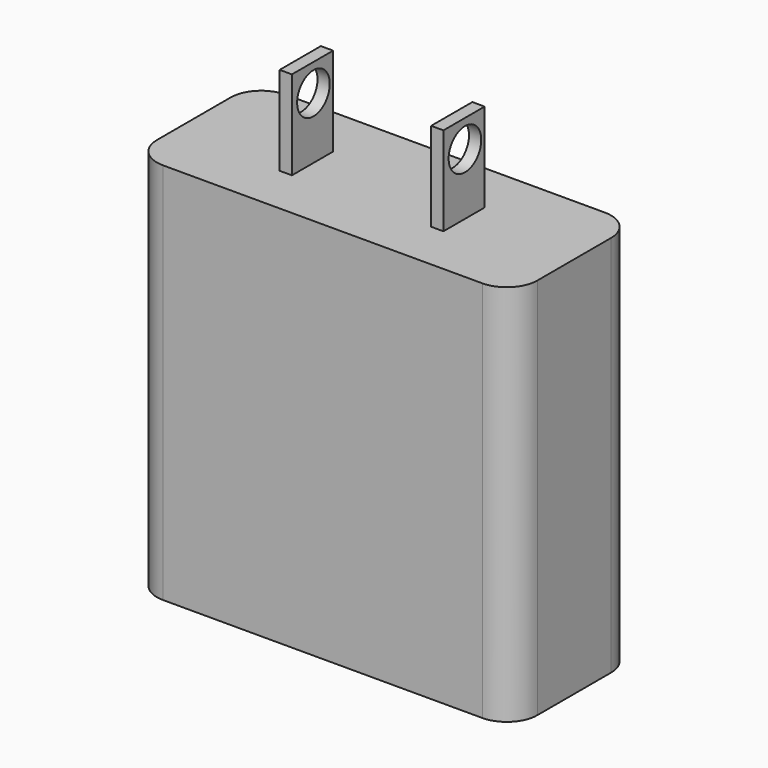
from build123d import *

# Parameters (mm, degrees)
F0_W      = 63.0582608283
F0_H      = 63.4325034916
F1_DEPTH  = 12.7
F2_R      = 5.08
F4_E1_W   = 8.5344002582
F4_E1_H   = 14.732
F5_DEPTH  = 2.032
F4_E2_W   = 8.5344002582
F4_E2_H   = 14.732
F6_DEPTH  = 2.032
F8_D      = 6.7564
F9_W      = 11.2923893612
F9_H      = 4.2961570434
F10_DEPTH = 7.112
F11_R     = 1.4717045876


with BuildPart() as f1:
    # F0 (on Front) → F1 (new body, symmetric)
    with BuildSketch(Plane.XZ):
        with Locations((-4.5010391623, -6.8866405636)):
            Rectangle(F0_W, F0_H)
    extrude(amount=F1_DEPTH, both=True)

    # F2
    f2_edges = [f1.edges().sort_by_distance(p)[0] for p in [
        (27.028091, -12.7, -6.886641),
        (27.028091, 12.7, -6.886641),
        (-36.03017, 12.7, -6.886641),
        (-36.03017, -12.7, -6.886641),
    ]]
    fillet(f2_edges, radius=F2_R)

    # F4_E1 (on explicit) → F5 (join)
    with BuildSketch(Plane(origin=(-16.1959640682, 4.0732366033, 24.8296111822), x_dir=(0, -1, 0), z_dir=(-1, 0, 0))):
        with Locations((4.2672001291, 7.366)):
            Rectangle(F4_E1_W, F4_E1_H)
    extrude(amount=F5_DEPTH)

    # F4_E2 (on explicit) → F6 (join)
    with BuildSketch(Plane(origin=(6.8857083097, 4.0732364287, 24.8296111822), x_dir=(0, -1, 0), z_dir=(-1, 0, 0))):
        with Locations((4.2672001291, 7.366)):
            Rectangle(F4_E2_W, F4_E2_H)
    extrude(amount=-F6_DEPTH)

    # F8 (through all)
    with Locations(Plane.YZ.offset(8.9177083097)):
        with Locations((0, 34.9955298007)):
            Hole(F8_D / 2)

    # F9 (on face) → F10 (cut)
    with BuildSketch(Plane(origin=(0, 0, -38.6028923094), x_dir=(1, 0, 0), z_dir=(0, 0, -1))):
        with Locations((-3.2546349103, 0.5336764734)):
            Rectangle(F9_W, F9_H)
    extrude(amount=-F10_DEPTH, mode=Mode.SUBTRACT)

    # F11
    f11_edges = [f1.edges().sort_by_distance(p)[0] for p in [
        (-8.90083, 1.614402, -35.046892),
    ]]
    fillet(f11_edges, radius=F11_R)


solid = f1.part
